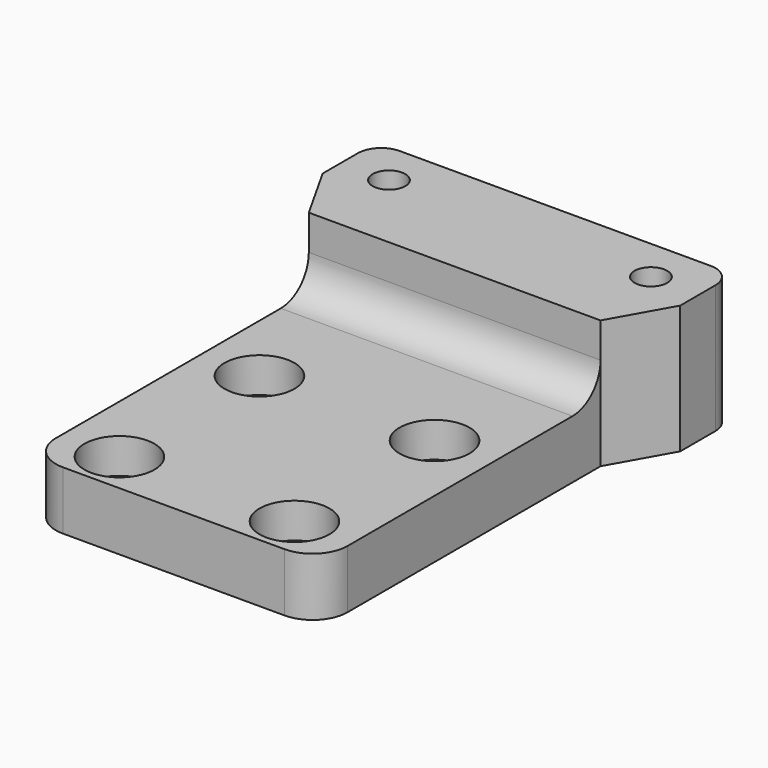
from build123d import *

# Parameters (mm, degrees)
F0_W     = 25
F0_H     = 30.0927665085
F0_W_2   = 30.6387297809
F0_H_2   = 5.7677225769
F1_DEPTH = 5
F2_R     = 1.675
F3_DEPTH = 25
F4_R     = 3
F5_DEPTH = 11
F6_R     = 1.4
F7_DEPTH = 11.001
F2_R_2   = 3
F8_DEPTH = 3
F9_R     = 3
F10_R    = 2


# Not quite as in the source:
# - a feature names something its author has since deleted; it is built from what else it names


with BuildPart() as f1:
    # F0 (on Top) → F1 (new body)
    with BuildSketch(Plane.XY):
        with Locations((12.5, 15.0463832542)):
            Rectangle(F0_W, F0_H)
        Polygon((-2.8193648905, 35.1040735841), (0, 30.0927665085), (25, 30.0927665085), (27.8193648905, 35.1040735841), align=None)
        with Locations((12.5, 37.9879348725)):
            Rectangle(F0_W_2, F0_H_2)
    extrude(amount=F1_DEPTH)

    # F2 (on face) → F3 (cut)
    with BuildSketch(Plane.XY.offset(5)):
        with BuildLine():
            ThreePointArc((3.325, 18.5605346784), (5, 16.8855346784), (6.675, 18.5605346784))
            ThreePointArc((6.675, 18.5605346784), (5, 20.2355346784), (3.325, 18.5605346784))
        make_face()
        with Locations((20, 18.5605346784)):
            Circle(F2_R)
        with Locations((20, 3.5605346784)):
            Circle(F2_R)
        with Locations((5, 3.5605346784)):
            Circle(F2_R)
    extrude(amount=-F3_DEPTH, mode=Mode.SUBTRACT)

    # F4
    f4_edges = [f1.edges().sort_by_distance(p)[0] for p in [
        (0, 0, 2.5),
        (25, 0, 2.5),
    ]]
    fillet(f4_edges, radius=F4_R)

    # F0 (on Top) → F5 (join)
    with BuildSketch(Plane.XY):
        with Locations((12.5, 37.9879348725)):
            Rectangle(F0_W_2, F0_H_2)
        Polygon((-2.8193648905, 35.1040735841), (0, 30.0927665085), (25, 30.0927665085), (27.8193648905, 35.1040735841), align=None)
    extrude(amount=F5_DEPTH)

    # F6 (on face) → F7 (cut, through all)
    with BuildSketch(Plane.XY.offset(11)):
        with Locations((23.6868802458, 37.1295362711)):
            Circle(F6_R)
        with BuildLine():
            ThreePointArc((-0.1581197542, 37.1295362711), (1.2418802458, 35.7295362711), (2.6418802458, 37.1295362711))
            ThreePointArc((2.6418802458, 37.1295362711), (1.2418802458, 38.5295362711), (-0.1581197542, 37.1295362711))
        make_face()
    extrude(amount=-F7_DEPTH, mode=Mode.SUBTRACT)

    # F2 (on face) → F8 (cut)
    with BuildSketch(Plane.XY.offset(5)):
        with BuildLine():
            ThreePointArc((8, 18.5605346784), (5, 21.5605346784), (2, 18.5605346784))
            ThreePointArc((2, 18.5605346784), (5, 15.5605346784), (8, 18.5605346784))
        make_face()
        with BuildLine():
            ThreePointArc((3.325, 18.5605346784), (5, 20.2355346784), (6.675, 18.5605346784))
            ThreePointArc((6.675, 18.5605346784), (5, 16.8855346784), (3.325, 18.5605346784))
        make_face(mode=Mode.SUBTRACT)
        with Locations((5, 3.5605346784)):
            Circle(F2_R_2)
        with Locations((5, 3.5605346784)):
            Circle(F2_R, mode=Mode.SUBTRACT)
        with Locations((20, 18.5605346784)):
            Circle(F2_R_2)
        with Locations((20, 18.5605346784)):
            Circle(F2_R, mode=Mode.SUBTRACT)
        with Locations((20, 3.5605346784)):
            Circle(F2_R_2)
        with Locations((20, 3.5605346784)):
            Circle(F2_R, mode=Mode.SUBTRACT)
    extrude(amount=-F8_DEPTH, mode=Mode.SUBTRACT)

    # F9
    f9_edges = [f1.edges().sort_by_distance(p)[0] for p in [
        (12.5, 30.092767, 5),
    ]]
    fillet(f9_edges, radius=F9_R)

    # F10
    f10_edges = [f1.edges().sort_by_distance(p)[0] for p in [
        (27.819365, 40.871796, 5.5),
        (-2.819365, 40.871796, 5.5),
    ]]
    fillet(f10_edges, radius=F10_R)


solid = f1.part
